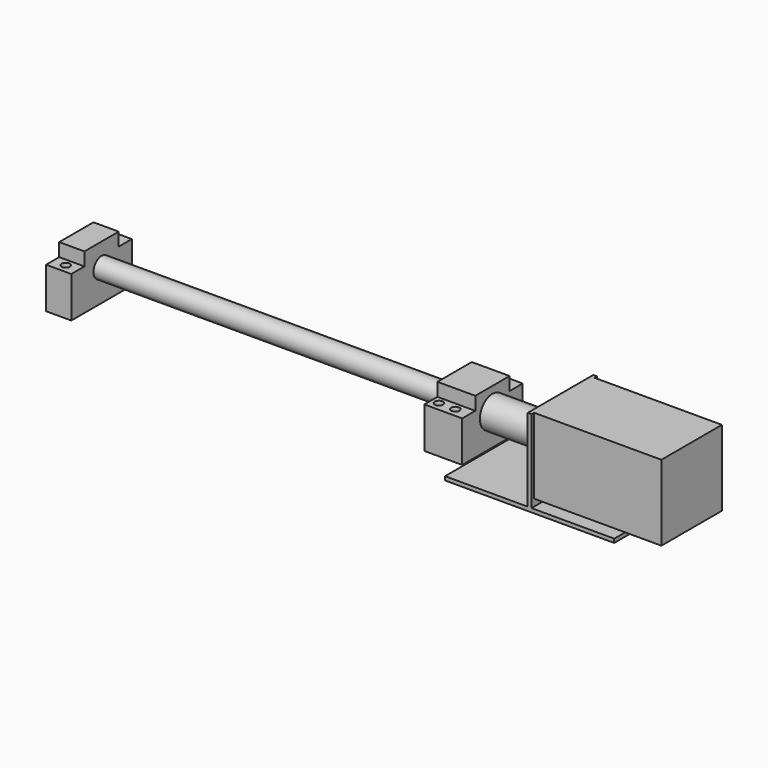
from build123d import *

# Parameters (mm, degrees)
F0_R      = 8
F1_DEPTH  = 330
F3_DEPTH  = 30
F5_DEPTH  = 20
F6_R      = 12.5
F7_DEPTH  = 57
F8_R      = 3.3
F9_DEPTH  = 43.001
F10_W     = 60
F10_H     = 60
F11_DEPTH = 101
F13_DEPTH = 32.5
F14_W     = 65.58
F14_H     = 3
F15_DEPTH = 65


# Not quite as in the source:
# - a feature names something its author has since deleted; it is built from what else it names


with BuildPart() as f1:
    # F0 (on Right) → F1 (new body)
    with BuildSketch(Plane.YZ):
        Circle(F0_R)
    extrude(amount=F1_DEPTH)

    # F2 (on face) → F3 (join)
    with BuildSketch(Plane.YZ.offset(330)):
        Polygon((30, 7.5), (17, 7.5), (17, 18), (-17, 18), (-17, 7.5), (-30, 7.5), (-30, -25), (30, -25), align=None)
    extrude(amount=-F3_DEPTH)

    # F4 (on face) → F5 (join)
    with BuildSketch(Plane(origin=(0, 0, 0), x_dir=(0, -1, 0), z_dir=(-1, 0, 0))):
        Polygon((17, 7.5), (17, 18), (-17, 18), (-17, 7.5), (-30, 7.5), (-30, -25), (30, -25), (30, 7.5), align=None)
    extrude(amount=-F5_DEPTH)

    # F6 (on face) → F7 (join)
    with BuildSketch(Plane.YZ.offset(330)):
        Circle(F6_R)
    extrude(amount=F7_DEPTH)

    # F8 (on face) → F9 (cut, through all)
    with BuildSketch(Plane.XY.offset(18)):
        with Locations((306, 23)):
            Circle(F8_R)
        with Locations((319, 23)):
            Circle(F8_R)
        with Locations((306, -23)):
            Circle(F8_R)
        with Locations((319, -23)):
            Circle(F8_R)
        with Locations((10, 23)):
            Circle(F8_R)
        with Locations((10, -23)):
            Circle(F8_R)
    extrude(amount=-F9_DEPTH, mode=Mode.SUBTRACT)

    # F10 (on face) → F11 (join)
    with BuildSketch(Plane.YZ.offset(387)):
        Rectangle(F10_W, F10_H)
    extrude(amount=F11_DEPTH)

    # F12 (on Front) → F13 (join, symmetric)
    with BuildSketch(Plane.XZ):
        Polygon((387, 30), (384, 30), (384, -38.58), (452.58, -38.58), (452.58, -35.58), (387, -35.58), align=None)
    extrude(amount=F13_DEPTH, both=True)

    # F14 (on face) → F15 (join, through all)
    with BuildSketch(Plane.XZ.offset(32.5)):
        with Locations((351.21, -37.08)):
            Rectangle(F14_W, F14_H)
    extrude(amount=-F15_DEPTH)


solid = f1.part
